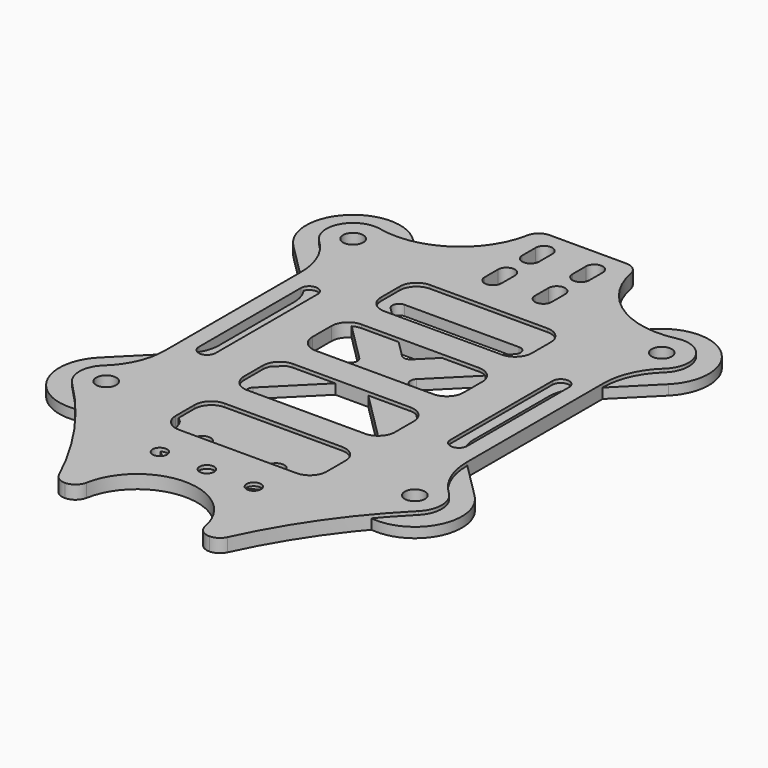
from build123d import *

# Parameters (mm, degrees)
F0_R        = 1.5
F0_R_2      = 1.525
F1_DEPTH    = 1.5
F2_DEPTH    = 1.5
F3_R        = 2.5
F4_R        = 1.075
F4_R_2      = 1.5
F5_DEPTH    = 2
F6_T1_DEPTH = 8.4667926391
F6_T3_DEPTH = 11.0807376097


# Not quite as in the source:
# - a fillet or chamfer that OpenCascade refuses, or shapes differently, is made with other operations: its cross-section is extruded or revolved along the edge and cut away or added


with BuildPart() as f1:
    # F0 (on Top) → F1 (new body)
    with BuildSketch(Plane.XY):
        with BuildLine():
            Line((-16.9705627485, 26.8700576851), (-18.0502525317, 27.9497474683))
            ThreePointArc((-18.0502525317, 27.9497474683), (-27.9497474683, 27.9497474683), (-27.9497474683, 18.0502525317))
            Line((-27.9497474683, 18.0502525317), (-20.4644660941, 10.5649711575))
            ThreePointArc((-20.4644660941, 10.5649711575), (-19.3806023374, 8.9428544133), (-19, 7.0294372515))
            Line((-19, 7.0294372515), (-19, -7.0294372515))
            ThreePointArc((-19, -7.0294372515), (-19.3806023374, -8.9428544133), (-20.4644660941, -10.5649711575))
            Line((-20.4644660941, -10.5649711575), (-27.9497474683, -18.0502525317))
            ThreePointArc((-27.9497474683, -18.0502525317), (-27.9497474683, -27.9497474683), (-18.0502525317, -27.9497474683))
            Line((-18.0502525317, -27.9497474683), (-16.9705627485, -26.8700576851))
            ThreePointArc((-16.9705627485, -26.8700576851), (-14.1541816284, -24.4586921902), (-11, -22.5098914259))
            ThreePointArc((-11, -22.5098914259), (0, -19.8406204336), (11, -22.5098914259))
            ThreePointArc((11, -22.5098914259), (14.1541816284, -24.4586921902), (16.9705627485, -26.8700576851))
            Line((16.9705627485, -26.8700576851), (18.0502525317, -27.9497474683))
            ThreePointArc((18.0502525317, -27.9497474683), (27.9497474683, -27.9497474683), (27.9497474683, -18.0502525317))
            Line((27.9497474683, -18.0502525317), (20.4644660941, -10.5649711575))
            ThreePointArc((20.4644660941, -10.5649711575), (19.3806023374, -8.9428544133), (19, -7.0294372515))
            Line((19, -7.0294372515), (19, 7.0294372515))
            ThreePointArc((19, 7.0294372515), (19.3806023374, 8.9428544133), (20.4644660941, 10.5649711575))
            Line((20.4644660941, 10.5649711575), (27.9497474683, 18.0502525317))
            ThreePointArc((27.9497474683, 18.0502525317), (27.9497474683, 27.9497474683), (18.0502525317, 27.9497474683))
            Line((18.0502525317, 27.9497474683), (16.9705627485, 26.8700576851))
            ThreePointArc((16.9705627485, 26.8700576851), (0, 19.8406204336), (-16.9705627485, 26.8700576851))
        make_face()
        with Locations((-23, -23)):
            Circle(F0_R, mode=Mode.SUBTRACT)
        with Locations((-15.25, -15.25)):
            Circle(F0_R_2, mode=Mode.SUBTRACT)
        with Locations((23, -23)):
            Circle(F0_R, mode=Mode.SUBTRACT)
        with BuildLine():
            ThreePointArc((-0.7071067812, -4.2426406871), (0, -3.9497474683), (0.7071067812, -4.2426406871))
            Line((0.7071067812, -4.2426406871), (9.2573593129, -12.7928932188))
            ThreePointArc((9.2573593129, -12.7928932188), (9.4741320642, -13.8826834324), (8.5502525317, -14.5))
            Line((8.5502525317, -14.5), (-8.5502525317, -14.5))
            ThreePointArc((-8.5502525317, -14.5), (-9.4741320642, -13.8826834324), (-9.2573593129, -12.7928932188))
            Line((-9.2573593129, -12.7928932188), (-0.7071067812, -4.2426406871))
        make_face(mode=Mode.SUBTRACT)
        with Locations((15.25, -15.25)):
            Circle(F0_R_2, mode=Mode.SUBTRACT)
        with BuildLine():
            ThreePointArc((-14.5, 8.5502525317), (-13.8826834324, 9.4741320642), (-12.7928932188, 9.2573593129))
            Line((-12.7928932188, 9.2573593129), (-4.2426406871, 0.7071067812))
            ThreePointArc((-4.2426406871, 0.7071067812), (-3.9497474683, 0), (-4.2426406871, -0.7071067812))
            Line((-4.2426406871, -0.7071067812), (-12.7928932188, -9.2573593129))
            ThreePointArc((-12.7928932188, -9.2573593129), (-13.8826834324, -9.4741320642), (-14.5, -8.5502525317))
            Line((-14.5, -8.5502525317), (-14.5, 8.5502525317))
        make_face(mode=Mode.SUBTRACT)
        with Locations((-15.25, 15.25)):
            Circle(F0_R_2, mode=Mode.SUBTRACT)
        with Locations((-23, 23)):
            Circle(F0_R, mode=Mode.SUBTRACT)
        with BuildLine():
            Line((12.7928932188, -9.2573593129), (4.2426406871, -0.7071067812))
            ThreePointArc((4.2426406871, -0.7071067812), (3.9497474683, 0), (4.2426406871, 0.7071067812))
            Line((4.2426406871, 0.7071067812), (12.7928932188, 9.2573593129))
            ThreePointArc((12.7928932188, 9.2573593129), (13.8826834324, 9.4741320642), (14.5, 8.5502525317))
            Line((14.5, 8.5502525317), (14.5, -8.5502525317))
            ThreePointArc((14.5, -8.5502525317), (13.8826834324, -9.4741320642), (12.7928932188, -9.2573593129))
        make_face(mode=Mode.SUBTRACT)
        with BuildLine():
            Line((-0.7071067812, 4.2426406871), (-9.2573593129, 12.7928932188))
            ThreePointArc((-9.2573593129, 12.7928932188), (-9.4741320642, 13.8826834324), (-8.5502525317, 14.5))
            Line((-8.5502525317, 14.5), (8.5502525317, 14.5))
            ThreePointArc((8.5502525317, 14.5), (9.4741320642, 13.8826834324), (9.2573593129, 12.7928932188))
            Line((9.2573593129, 12.7928932188), (0.7071067812, 4.2426406871))
            ThreePointArc((0.7071067812, 4.2426406871), (0, 3.9497474683), (-0.7071067812, 4.2426406871))
        make_face(mode=Mode.SUBTRACT)
        with Locations((15.25, 15.25)):
            Circle(F0_R_2, mode=Mode.SUBTRACT)
        with Locations((23, 23)):
            Circle(F0_R, mode=Mode.SUBTRACT)
    extrude(amount=F1_DEPTH)


with BuildPart() as f2:
    # F0 (on Top) → F2 (new body)
    with BuildSketch(Plane.XY):
        with BuildLine():
            Line((-16.9705627485, 26.8700576851), (-18.0502525317, 27.9497474683))
            ThreePointArc((-18.0502525317, 27.9497474683), (-27.9497474683, 27.9497474683), (-27.9497474683, 18.0502525317))
            Line((-27.9497474683, 18.0502525317), (-20.4644660941, 10.5649711575))
            ThreePointArc((-20.4644660941, 10.5649711575), (-19.3806023374, 8.9428544133), (-19, 7.0294372515))
            Line((-19, 7.0294372515), (-19, -7.0294372515))
            ThreePointArc((-19, -7.0294372515), (-19.3806023374, -8.9428544133), (-20.4644660941, -10.5649711575))
            Line((-20.4644660941, -10.5649711575), (-27.9497474683, -18.0502525317))
            ThreePointArc((-27.9497474683, -18.0502525317), (-27.9497474683, -27.9497474683), (-18.0502525317, -27.9497474683))
            Line((-18.0502525317, -27.9497474683), (-16.9705627485, -26.8700576851))
            ThreePointArc((-16.9705627485, -26.8700576851), (-14.1541816284, -24.4586921902), (-11, -22.5098914259))
            ThreePointArc((-11, -22.5098914259), (0, -19.8406204336), (11, -22.5098914259))
            ThreePointArc((11, -22.5098914259), (14.1541816284, -24.4586921902), (16.9705627485, -26.8700576851))
            Line((16.9705627485, -26.8700576851), (18.0502525317, -27.9497474683))
            ThreePointArc((18.0502525317, -27.9497474683), (27.9497474683, -27.9497474683), (27.9497474683, -18.0502525317))
            Line((27.9497474683, -18.0502525317), (20.4644660941, -10.5649711575))
            ThreePointArc((20.4644660941, -10.5649711575), (19.3806023374, -8.9428544133), (19, -7.0294372515))
            Line((19, -7.0294372515), (19, 7.0294372515))
            ThreePointArc((19, 7.0294372515), (19.3806023374, 8.9428544133), (20.4644660941, 10.5649711575))
            Line((20.4644660941, 10.5649711575), (27.9497474683, 18.0502525317))
            ThreePointArc((27.9497474683, 18.0502525317), (27.9497474683, 27.9497474683), (18.0502525317, 27.9497474683))
            Line((18.0502525317, 27.9497474683), (16.9705627485, 26.8700576851))
            ThreePointArc((16.9705627485, 26.8700576851), (0, 19.8406204336), (-16.9705627485, 26.8700576851))
        make_face()
        with Locations((-23, -23)):
            Circle(F0_R, mode=Mode.SUBTRACT)
        with Locations((-15.25, -15.25)):
            Circle(F0_R_2, mode=Mode.SUBTRACT)
        with Locations((23, -23)):
            Circle(F0_R, mode=Mode.SUBTRACT)
        with BuildLine():
            ThreePointArc((-0.7071067812, -4.2426406871), (0, -3.9497474683), (0.7071067812, -4.2426406871))
            Line((0.7071067812, -4.2426406871), (9.2573593129, -12.7928932188))
            ThreePointArc((9.2573593129, -12.7928932188), (9.4741320642, -13.8826834324), (8.5502525317, -14.5))
            Line((8.5502525317, -14.5), (-8.5502525317, -14.5))
            ThreePointArc((-8.5502525317, -14.5), (-9.4741320642, -13.8826834324), (-9.2573593129, -12.7928932188))
            Line((-9.2573593129, -12.7928932188), (-0.7071067812, -4.2426406871))
        make_face(mode=Mode.SUBTRACT)
        with Locations((15.25, -15.25)):
            Circle(F0_R_2, mode=Mode.SUBTRACT)
        with BuildLine():
            ThreePointArc((-14.5, 8.5502525317), (-13.8826834324, 9.4741320642), (-12.7928932188, 9.2573593129))
            Line((-12.7928932188, 9.2573593129), (-4.2426406871, 0.7071067812))
            ThreePointArc((-4.2426406871, 0.7071067812), (-3.9497474683, 0), (-4.2426406871, -0.7071067812))
            Line((-4.2426406871, -0.7071067812), (-12.7928932188, -9.2573593129))
            ThreePointArc((-12.7928932188, -9.2573593129), (-13.8826834324, -9.4741320642), (-14.5, -8.5502525317))
            Line((-14.5, -8.5502525317), (-14.5, 8.5502525317))
        make_face(mode=Mode.SUBTRACT)
        with Locations((-15.25, 15.25)):
            Circle(F0_R_2, mode=Mode.SUBTRACT)
        with Locations((-23, 23)):
            Circle(F0_R, mode=Mode.SUBTRACT)
        with BuildLine():
            Line((12.7928932188, -9.2573593129), (4.2426406871, -0.7071067812))
            ThreePointArc((4.2426406871, -0.7071067812), (3.9497474683, 0), (4.2426406871, 0.7071067812))
            Line((4.2426406871, 0.7071067812), (12.7928932188, 9.2573593129))
            ThreePointArc((12.7928932188, 9.2573593129), (13.8826834324, 9.4741320642), (14.5, 8.5502525317))
            Line((14.5, 8.5502525317), (14.5, -8.5502525317))
            ThreePointArc((14.5, -8.5502525317), (13.8826834324, -9.4741320642), (12.7928932188, -9.2573593129))
        make_face(mode=Mode.SUBTRACT)
        with BuildLine():
            Line((-0.7071067812, 4.2426406871), (-9.2573593129, 12.7928932188))
            ThreePointArc((-9.2573593129, 12.7928932188), (-9.4741320642, 13.8826834324), (-8.5502525317, 14.5))
            Line((-8.5502525317, 14.5), (8.5502525317, 14.5))
            ThreePointArc((8.5502525317, 14.5), (9.4741320642, 13.8826834324), (9.2573593129, 12.7928932188))
            Line((9.2573593129, 12.7928932188), (0.7071067812, 4.2426406871))
            ThreePointArc((0.7071067812, 4.2426406871), (0, 3.9497474683), (-0.7071067812, 4.2426406871))
        make_face(mode=Mode.SUBTRACT)
        with Locations((15.25, 15.25)):
            Circle(F0_R_2, mode=Mode.SUBTRACT)
        with Locations((23, 23)):
            Circle(F0_R, mode=Mode.SUBTRACT)
        with BuildLine():
            ThreePointArc((11, -22.5098914259), (0, -19.8406204336), (-11, -22.5098914259))
            Line((-11, -22.5098914259), (-9.0054434737, -29.8166890196))
            ThreePointArc((-9.0054434737, -29.8166890196), (-7.2164394139, -32.4738800371), (-4.1819250457, -33.5))
            Line((-4.1819250457, -33.5), (4.1819250457, -33.5))
            ThreePointArc((4.1819250457, -33.5), (7.2164394139, -32.4738800371), (9.0054434737, -29.8166890196))
            Line((9.0054434737, -29.8166890196), (11, -22.5098914259))
        make_face()
        with BuildLine():
            Line((-6.75, -29.5), (-6.75, -27))
            ThreePointArc((-6.75, -27), (-5.5, -25.75), (-4.25, -27))
            Line((-4.25, -27), (-4.25, -29.5))
            ThreePointArc((-4.25, -29.5), (-5.5, -30.75), (-6.75, -29.5))
        make_face(mode=Mode.SUBTRACT)
        with BuildLine():
            ThreePointArc((4.25, -27), (5.5, -25.75), (6.75, -27))
            Line((6.75, -27), (6.75, -29.5))
            ThreePointArc((6.75, -29.5), (5.5, -30.75), (4.25, -29.5))
            Line((4.25, -29.5), (4.25, -27))
        make_face(mode=Mode.SUBTRACT)
    extrude(amount=F2_DEPTH)

    # F3
    f3_edges = [f2.edges().sort_by_distance(p)[0] for p in [
        (-11, -22.509891, 0.75),
        (11, -22.509891, 0.75),
    ]]
    fillet(f3_edges, radius=F3_R)


with BuildPart() as f5:
    # F4 (on Top) → F5 (new body)
    with BuildSketch(Plane.XY):
        with BuildLine():
            ThreePointArc((-25.7142857143, 20.0618623141), (-23.3387461869, 16.7254367281), (-22.5, 12.7165180994))
            Line((-22.5, 12.7165180994), (-22.5, 0))
            Line((-22.5, 0), (-22.5, -12.7165180994))
            ThreePointArc((-22.5, -12.7165180994), (-23.3387461869, -16.7254367281), (-25.7142857143, -20.0618623141))
            ThreePointArc((-25.7142857143, -20.0618623141), (-26.9992166524, -22.9208408742), (-25.8284271247, -25.8284271247))
            ThreePointArc((-25.8284271247, -25.8284271247), (-17.9985525415, -35.2710579181), (-12.0521238575, -46))
            Line((-12.0521238575, -46), (-8.9702131196, -46))
            ThreePointArc((-8.9702131196, -46), (0, -37.0297868804), (8.9702131196, -46))
            Line((8.9702131196, -46), (12.0521238575, -46))
            ThreePointArc((12.0521238575, -46), (17.9985525415, -35.2710579181), (25.8284271247, -25.8284271247))
            ThreePointArc((25.8284271247, -25.8284271247), (26.9992166524, -22.9208408742), (25.7142857143, -20.0618623141))
            ThreePointArc((25.7142857143, -20.0618623141), (23.3387461869, -16.7254367281), (22.5, -12.7165180994))
            Line((22.5, -12.7165180994), (22.5, 0))
            Line((22.5, 0), (22.5, 12.7165180994))
            ThreePointArc((22.5, 12.7165180994), (23.3387461869, 16.7254367281), (25.7142857143, 20.0618623141))
            ThreePointArc((25.7142857143, 20.0618623141), (26.5411769878, 24.8601251413), (22.1211339094, 26.9022550397))
            ThreePointArc((22.1211339094, 26.9022550397), (12.899127204, 28.5774502036), (7.6947540906, 36.3727171655))
            ThreePointArc((7.6947540906, 36.3727171655), (7.005440465, 37.5403626734), (5.7297904995, 38))
            Line((5.7297904995, 38), (-5.7297904995, 38))
            ThreePointArc((-5.7297904995, 38), (-7.005440465, 37.5403626734), (-7.6947540906, 36.3727171655))
            ThreePointArc((-7.6947540906, 36.3727171655), (-12.899127204, 28.5774502036), (-22.1211339094, 26.9022550397))
            ThreePointArc((-22.1211339094, 26.9022550397), (-26.5411769878, 24.8601251413), (-25.7142857143, 20.0618623141))
        make_face()
        with Locations((-7, -33)):
            Circle(F4_R, mode=Mode.SUBTRACT)
        with Locations((-23, -23)):
            Circle(F4_R_2, mode=Mode.SUBTRACT)
        with Locations((0, -33)):
            Circle(F4_R, mode=Mode.SUBTRACT)
        with Locations((7, -33)):
            Circle(F4_R, mode=Mode.SUBTRACT)
        with BuildLine():
            Line((-11.25, -24.75), (-11.25, -21.25))
            ThreePointArc((-11.25, -21.25), (-10.517766953, -19.482233047), (-8.75, -18.75))
            Line((-8.75, -18.75), (8.75, -18.75))
            ThreePointArc((8.75, -18.75), (10.517766953, -19.482233047), (11.25, -21.25))
            Line((11.25, -21.25), (11.25, -24.75))
            ThreePointArc((11.25, -24.75), (10.517766953, -26.517766953), (8.75, -27.25))
            Line((8.75, -27.25), (-8.75, -27.25))
            ThreePointArc((-8.75, -27.25), (-10.517766953, -26.517766953), (-11.25, -24.75))
        make_face(mode=Mode.SUBTRACT)
        with BuildLine():
            Line((-11.25, -12), (-11.25, -8.5))
            ThreePointArc((-11.25, -8.5), (-10.517766953, -6.732233047), (-8.75, -6))
            Line((-8.75, -6), (8.75, -6))
            ThreePointArc((8.75, -6), (10.517766953, -6.732233047), (11.25, -8.5))
            Line((11.25, -8.5), (11.25, -12))
            ThreePointArc((11.25, -12), (10.517766953, -13.767766953), (8.75, -14.5))
            Line((8.75, -14.5), (-8.75, -14.5))
            ThreePointArc((-8.75, -14.5), (-10.517766953, -13.767766953), (-11.25, -12))
        make_face(mode=Mode.SUBTRACT)
        with Locations((23, -23)):
            Circle(F4_R_2, mode=Mode.SUBTRACT)
        with BuildLine():
            Line((-20, -9.5), (-20, 9.5))
            ThreePointArc((-20, 9.5), (-18.75, 10.75), (-17.5, 9.5))
            Line((-17.5, 9.5), (-17.5, -9.5))
            ThreePointArc((-17.5, -9.5), (-18.75, -10.75), (-20, -9.5))
        make_face(mode=Mode.SUBTRACT)
        with Locations((-23, 23)):
            Circle(F4_R_2, mode=Mode.SUBTRACT)
        with BuildLine():
            Line((-5, 25), (-5, 27.5))
            ThreePointArc((-5, 27.5), (-3.75, 28.75), (-2.5, 27.5))
            Line((-2.5, 27.5), (-2.5, 25))
            ThreePointArc((-2.5, 25), (-3.75, 23.75), (-5, 25))
        make_face(mode=Mode.SUBTRACT)
        with BuildLine():
            ThreePointArc((-5, 34.5), (-3.75, 35.75), (-2.5, 34.5))
            Line((-2.5, 34.5), (-2.5, 32))
            ThreePointArc((-2.5, 32), (-3.75, 30.75), (-5, 32))
            Line((-5, 32), (-5, 34.5))
        make_face(mode=Mode.SUBTRACT)
        with BuildLine():
            Line((-11.25, 0.75), (-11.25, 4.25))
            ThreePointArc((-11.25, 4.25), (-10.517766953, 6.017766953), (-8.75, 6.75))
            Line((-8.75, 6.75), (8.75, 6.75))
            ThreePointArc((8.75, 6.75), (10.517766953, 6.017766953), (11.25, 4.25))
            Line((11.25, 4.25), (11.25, 0.75))
            ThreePointArc((11.25, 0.75), (10.517766953, -1.017766953), (8.75, -1.75))
            Line((8.75, -1.75), (-8.75, -1.75))
            ThreePointArc((-8.75, -1.75), (-10.517766953, -1.017766953), (-11.25, 0.75))
        make_face(mode=Mode.SUBTRACT)
        with BuildLine():
            ThreePointArc((-11.25, 17), (-10.517766953, 18.767766953), (-8.75, 19.5))
            Line((-8.75, 19.5), (8.75, 19.5))
            ThreePointArc((8.75, 19.5), (10.517766953, 18.767766953), (11.25, 17))
            Line((11.25, 17), (11.25, 13.5))
            ThreePointArc((11.25, 13.5), (10.517766953, 11.732233047), (8.75, 11))
            Line((8.75, 11), (-8.75, 11))
            ThreePointArc((-8.75, 11), (-10.517766953, 11.732233047), (-11.25, 13.5))
            Line((-11.25, 13.5), (-11.25, 17))
        make_face(mode=Mode.SUBTRACT)
        with BuildLine():
            Line((17.5, -9.5), (17.5, 9.5))
            ThreePointArc((17.5, 9.5), (18.75, 10.75), (20, 9.5))
            Line((20, 9.5), (20, -9.5))
            ThreePointArc((20, -9.5), (18.75, -10.75), (17.5, -9.5))
        make_face(mode=Mode.SUBTRACT)
        with BuildLine():
            ThreePointArc((2.5, 27.5), (3.75, 28.75), (5, 27.5))
            Line((5, 27.5), (5, 25))
            ThreePointArc((5, 25), (3.75, 23.75), (2.5, 25))
            Line((2.5, 25), (2.5, 27.5))
        make_face(mode=Mode.SUBTRACT)
        with BuildLine():
            ThreePointArc((5, 32), (3.75, 30.75), (2.5, 32))
            Line((2.5, 32), (2.5, 34.5))
            ThreePointArc((2.5, 34.5), (3.75, 35.75), (5, 34.5))
            Line((5, 34.5), (5, 32))
        make_face(mode=Mode.SUBTRACT)
        with Locations((23, 23)):
            Circle(F4_R_2, mode=Mode.SUBTRACT)
    extrude(amount=F5_DEPTH)

    # F6: fillet of radius 2 on 4 edges, made by hand

    # F6_s2 → F6_t1 (cut)
    with BuildSketch(Plane.XY.offset(-3.2333963195)):
        with BuildLine():
            ThreePointArc((-10.7587653296, -46), (-11.8367574682, -45.6846165585), (-12.5747687362, -44.8379329491))
            ThreePointArc((-12.5747687362, -44.8379329491), (-12.3106407447, -45.4177046649), (-12.0521238575, -46))
            Line((-12.0521238575, -46), (-10.7587653296, -46))
        make_face()
        with BuildLine():
            ThreePointArc((12.5747687362, -44.8379329491), (11.8367574682, -45.6846165585), (10.7587653296, -46))
            Line((10.7587653296, -46), (12.0521238575, -46))
            ThreePointArc((12.0521238575, -46), (12.3106407447, -45.4177046649), (12.5747687362, -44.8379329491))
        make_face()
    extrude(amount=F6_T1_DEPTH, mode=Mode.SUBTRACT)

    # F6_s4 → F6_t3 (cut)
    with BuildSketch(Plane.XY.offset(-4.5403688049)):
        with BuildLine():
            ThreePointArc((-8.8198791295, -44.3646237276), (-9.5075423306, -45.5377333083), (-10.7863606416, -46))
            Line((-10.7863606416, -46), (-8.9702131196, -46))
            ThreePointArc((-8.9702131196, -46), (-8.9325505566, -45.1788642224), (-8.8198791295, -44.3646237276))
        make_face()
        with BuildLine():
            ThreePointArc((10.7863606416, -46), (9.5075423306, -45.5377333083), (8.8198791295, -44.3646237276))
            ThreePointArc((8.8198791295, -44.3646237276), (8.9325505566, -45.1788642224), (8.9702131196, -46))
            Line((8.9702131196, -46), (10.7863606416, -46))
        make_face()
    extrude(amount=F6_T3_DEPTH, mode=Mode.SUBTRACT)


solid = Compound([f1.part, f2.part, f5.part])
